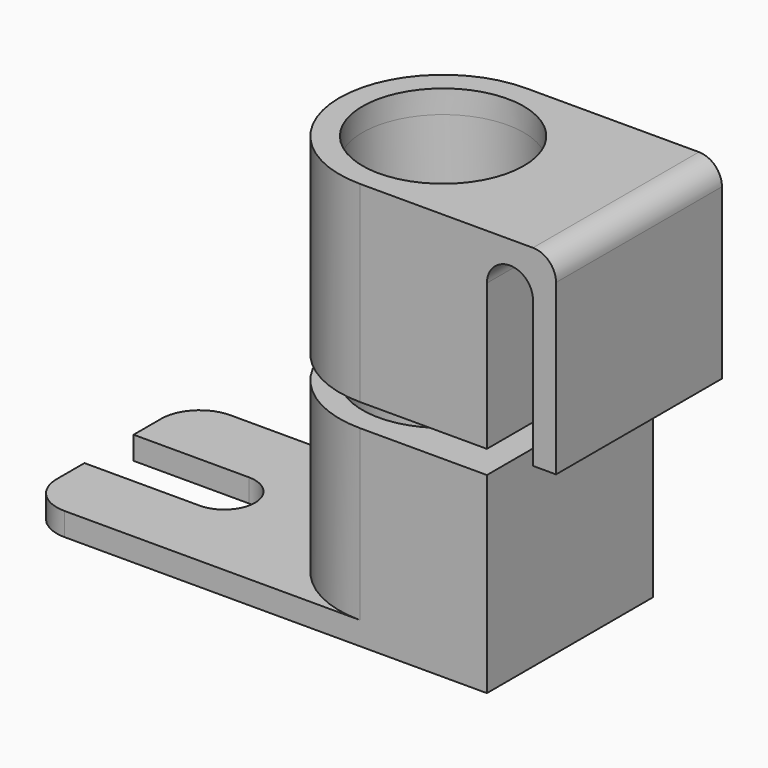
from build123d import *

# Parameters (mm, degrees)
F0_R     = 10.5
F0_W     = 6
F0_H     = 27
F0_W_2   = 3
F1_DEPTH = 3
F2_DEPTH = 22
F3_R     = 2.99999
F5_R     = 10.5
F6_DEPTH = 22
F7_DEPTH = 3
F8_R     = 5


# Not quite as in the source:
# - a fillet or chamfer is up to 0.001 mm smaller than in the source, because OpenCascade refuses the exact size


with BuildPart() as f1:
    # F0 (on Top) → F1 (new body)
    with BuildSketch(Plane.XY):
        with BuildLine():
            ThreePointArc((0, -13.5), (9.545941546, -9.545941546), (13.5, 0))
            ThreePointArc((13.5, 0), (9.545941546, 9.545941546), (0, 13.5))
            ThreePointArc((0, 13.5), (-13.5, 0), (0, -13.5))
        make_face()
        Circle(F0_R, mode=Mode.SUBTRACT)
        with BuildLine():
            Line((13.5, -13.5), (13.5, 0))
            ThreePointArc((13.5, 0), (9.545941546, -9.545941546), (0, -13.5))
            Line((0, -13.5), (13.5, -13.5))
        make_face()
        with BuildLine():
            ThreePointArc((0, 13.5), (9.545941546, 9.545941546), (13.5, 0))
            Line((13.5, 0), (13.5, 13.5))
            Line((13.5, 13.5), (0, 13.5))
        make_face()
        Polygon((13.5, 13.5), (13.5, 0), (13.5, -13.5), (16.5, -13.5), (16.5, 13.5), align=None)
        with Locations((19.5, 0)):
            Rectangle(F0_W, F0_H)
        with Locations((24, 0)):
            Rectangle(F0_W_2, F0_H)
    extrude(amount=F1_DEPTH)

    # F0 (on Top) → F2 (join)
    with BuildSketch(Plane.XY):
        with BuildLine():
            ThreePointArc((0, -13.5), (9.545941546, -9.545941546), (13.5, 0))
            ThreePointArc((13.5, 0), (9.545941546, 9.545941546), (0, 13.5))
            ThreePointArc((0, 13.5), (-13.5, 0), (0, -13.5))
        make_face()
        Circle(F0_R, mode=Mode.SUBTRACT)
        with BuildLine():
            ThreePointArc((0, 13.5), (9.545941546, 9.545941546), (13.5, 0))
            Line((13.5, 0), (13.5, 13.5))
            Line((13.5, 13.5), (0, 13.5))
        make_face()
        Polygon((13.5, 13.5), (13.5, 0), (13.5, -13.5), (16.5, -13.5), (16.5, 13.5), align=None)
        with Locations((24, 0)):
            Rectangle(F0_W_2, F0_H)
        with BuildLine():
            Line((13.5, -13.5), (13.5, 0))
            ThreePointArc((13.5, 0), (9.545941546, -9.545941546), (0, -13.5))
            Line((0, -13.5), (13.5, -13.5))
        make_face()
    extrude(amount=-F2_DEPTH)

    # F3 (radius 3 in the source; OpenCascade refuses exactly that, so slightly less here)
    f3_edges = [f1.edges().sort_by_distance(p)[0] for p in [
        (16.5, 0, 0),
        (22.5, 0, 0),
        (25.5, 0, 3),
    ]]
    fillet(f3_edges, radius=F3_R)


with BuildPart() as f6:
    # F5 (on offset) → F6 (new body)
    with BuildSketch(Plane(origin=(0, 0, -47), x_dir=(1, 0, 0), z_dir=(0, 0, -1))):
        with BuildLine():
            Line((16.5, 13.5), (0, 13.5))
            ThreePointArc((0, 13.5), (-13.5, 0), (0, -13.5))
            Line((0, -13.5), (16.5, -13.5))
            Line((16.5, -13.5), (16.5, 13.5))
        make_face()
        Circle(F5_R, mode=Mode.SUBTRACT)
    extrude(amount=-F6_DEPTH)

    # F5 (on offset) → F7 (join)
    with BuildSketch(Plane(origin=(0, 0, -47), x_dir=(1, 0, 0), z_dir=(0, 0, -1))):
        with BuildLine():
            Line((16.5, 13.5), (0, 13.5))
            ThreePointArc((0, 13.5), (-13.5, 0), (0, -13.5))
            Line((0, -13.5), (16.5, -13.5))
            Line((16.5, -13.5), (16.5, 13.5))
        make_face()
        Circle(F5_R, mode=Mode.SUBTRACT)
        with BuildLine():
            ThreePointArc((0, -13.5), (-13.5, 0), (0, 13.5))
            Line((0, 13.5), (-43.5, 13.5))
            Line((-43.5, 13.5), (-43.5, 4))
            Line((-43.5, 4), (-28.5, 4))
            ThreePointArc((-28.5, 4), (-24.5, 0), (-28.5, -4))
            Line((-28.5, -4), (-43.5, -4))
            Line((-43.5, -4), (-43.5, -13.5))
            Line((-43.5, -13.5), (0, -13.5))
        make_face()
    extrude(amount=F7_DEPTH)

    # F8
    f8_edges = [f6.edges().sort_by_distance(p)[0] for p in [
        (-43.5, -13.5, -48.5),
        (-43.5, 13.5, -48.5),
    ]]
    fillet(f8_edges, radius=F8_R)


solid = Compound([f1.part, f6.part])
